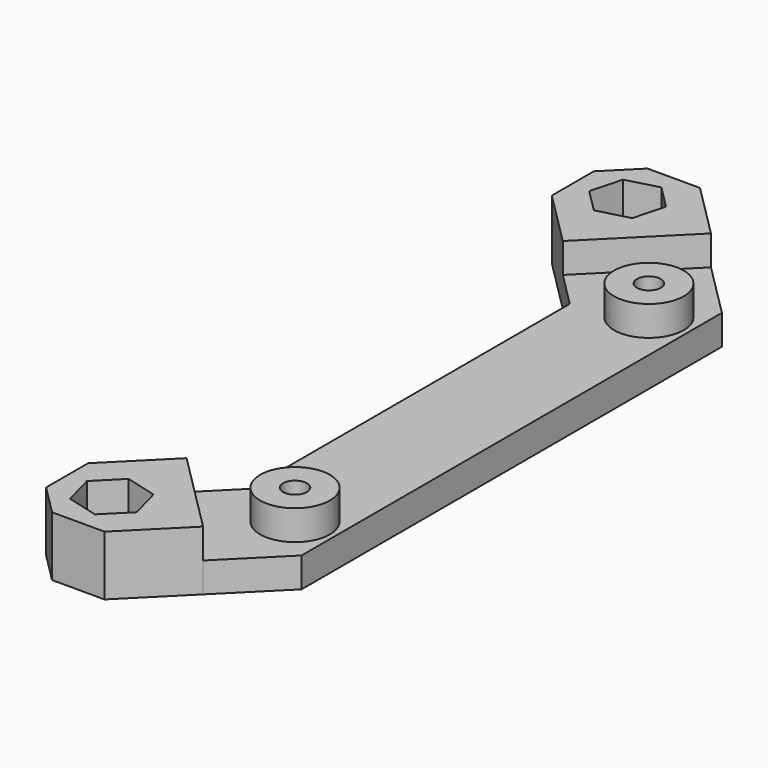
from build123d import *

# Parameters (mm, degrees)
F0_W     = 19.275
F0_H     = 74.8
F0_R     = 1.75
F0_R_2   = 1.2
F1_DEPTH = 6
F3_DEPTH = 25
F2_R     = 1.2
F4_DEPTH = 3
F5_SIZE  = 3
F2_R_2   = 1.75
F6_DEPTH = 4
F7_R     = 3.5
F7_R_2   = 1.2
F8_DEPTH = 3


# Not quite as in the source:
# - a feature names something its author has since deleted; it is built from what else it names


with BuildPart() as f1:
    # F0 (on Top) → F1 (new body)
    with BuildSketch(Plane.XY):
        with Locations((-45.9428956378, 11.8681262247)):
            Rectangle(F0_W, F0_H)
        with Locations((-50.5803956378, -20.5318737753)):
            Circle(F0_R, mode=Mode.SUBTRACT)
        with Locations((-40.3053956378, -10.3568737753)):
            Circle(F0_R_2, mode=Mode.SUBTRACT)
        with Locations((-40.3053956378, 34.0931262247)):
            Circle(F0_R_2, mode=Mode.SUBTRACT)
        with Locations((-50.5803956378, 44.2681262247)):
            Circle(F0_R, mode=Mode.SUBTRACT)
    extrude(amount=F1_DEPTH)

    # F2 (on face) → F3 (cut)
    with BuildSketch(Plane.XY.offset(6)):
        Polygon((-47.307246298, 49.2681262247), (-41.8063209679, 43.7672008947), (-36.3053956378, 38.2662755646), (-36.3053956378, 49.2681262247), align=None)
        Polygon((-55.5803956378, 40.9949768848), (-55.5803956378, -17.2587244354), (-50.0794703078, -11.7577991053), (-46.5803956378, -8.2587244354), (-46.5803956378, 31.9949768848), (-50.0794703078, 35.4940515548), align=None)
        Polygon((-36.3053956378, -14.5300231152), (-41.8063209679, -20.0309484452), (-47.307246298, -25.5318737753), (-36.3053956378, -25.5318737753), align=None)
    extrude(amount=-F3_DEPTH, mode=Mode.SUBTRACT)

    # F2 (on face) → F4 (cut)
    with BuildSketch(Plane.XY.offset(6)):
        Polygon((-46.5803956378, -8.2587244354), (-50.0794703078, -11.7577991053), (-41.8063209679, -20.0309484452), (-36.3053956378, -14.5300231152), (-36.3053956378, 38.2662755646), (-41.8063209679, 43.7672008947), (-50.0794703078, 35.4940515548), (-46.5803956378, 31.9949768848), align=None)
        with Locations((-40.3053956378, -10.3568737753)):
            Circle(F2_R, mode=Mode.SUBTRACT)
        with Locations((-40.3053956378, 34.0931262247)):
            Circle(F2_R, mode=Mode.SUBTRACT)
    extrude(amount=-F4_DEPTH, mode=Mode.SUBTRACT)

    # F5
    f5_edges = [f1.edges().sort_by_distance(p)[0] for p in [
        (-55.580396, 49.268126, 3),
        (-55.580396, -25.531874, 3),
    ]]
    chamfer(f5_edges, length=F5_SIZE)

    # F2 (on face) → F6 (cut)
    with BuildSketch(Plane.XY.offset(6)):
        Polygon((-49.7286489393, 47.4468881789), (-52.9074108935, 46.5951414804), (-53.759157592, 43.4163795262), (-51.4321423364, 41.0893642705), (-48.2533803822, 41.9411109691), (-47.4016336836, 45.1198729233), align=None)
        with Locations((-50.5803956378, 44.2681262247)):
            Circle(F2_R_2, mode=Mode.SUBTRACT)
        Polygon((-52.9074108935, -22.8588890309), (-49.7286489393, -23.7106357295), (-47.4016336836, -21.3836204738), (-48.2533803822, -18.2048585196), (-51.4321423364, -17.3531118211), (-53.759157592, -19.6801270767), align=None)
        with Locations((-50.5803956378, -20.5318737753)):
            Circle(F2_R_2, mode=Mode.SUBTRACT)
    extrude(amount=-F6_DEPTH, mode=Mode.SUBTRACT)

    # F7 (on face) → F8 (join)
    with BuildSketch(Plane.XY.offset(3)):
        with Locations((-40.3053956378, -10.3568737753)):
            Circle(F7_R)
        with Locations((-40.3053956378, -10.3568737753)):
            Circle(F7_R_2, mode=Mode.SUBTRACT)
        with Locations((-40.3053956378, 34.0931262247)):
            Circle(F7_R)
        with Locations((-40.3053956378, 34.0931262247)):
            Circle(F7_R_2, mode=Mode.SUBTRACT)
    extrude(amount=F8_DEPTH)


solid = f1.part
